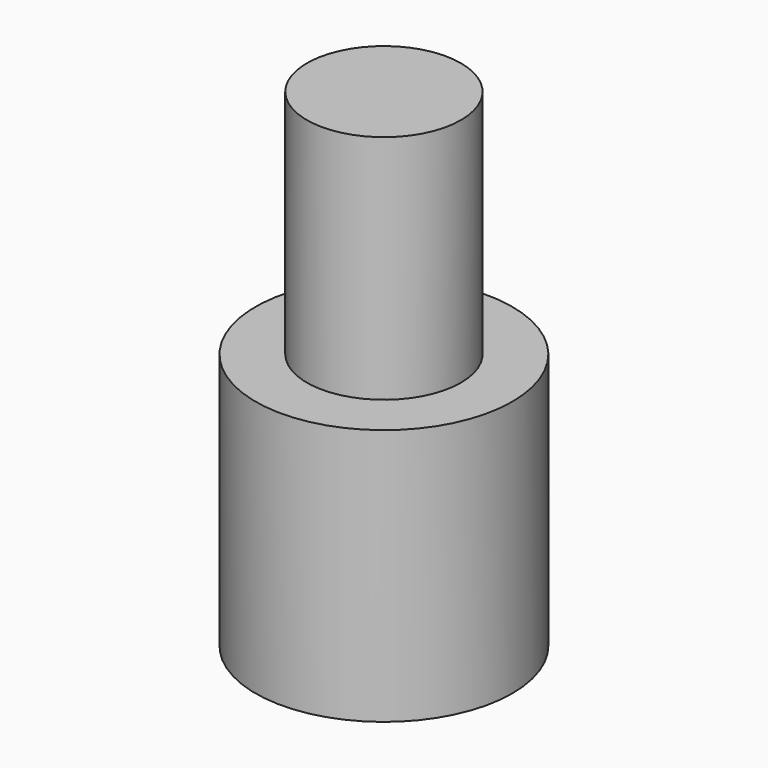
from build123d import *

# Parameters (mm, degrees)
F0_R     = 1.5
F0_R_2   = 0.5
F1_DEPTH = 4.5
F2_R     = 2.5
F2_R_2   = 1.5
F3_DEPTH = 5


with BuildPart() as f1:
    # F0 (on Top) → F1 (new body)
    with BuildSketch(Plane.XY):
        Circle(F0_R)
        Circle(F0_R_2, mode=Mode.SUBTRACT)
        Circle(F0_R_2)
    extrude(amount=-F1_DEPTH)

    # F2 (on face) → F3 (join)
    with BuildSketch(Plane(origin=(0, 0, -4.5), x_dir=(1, 0, 0), z_dir=(0, 0, -1))):
        Circle(F2_R)
        Circle(F2_R_2, mode=Mode.SUBTRACT)
        Circle(F2_R_2)
    extrude(amount=F3_DEPTH)


solid = f1.part
